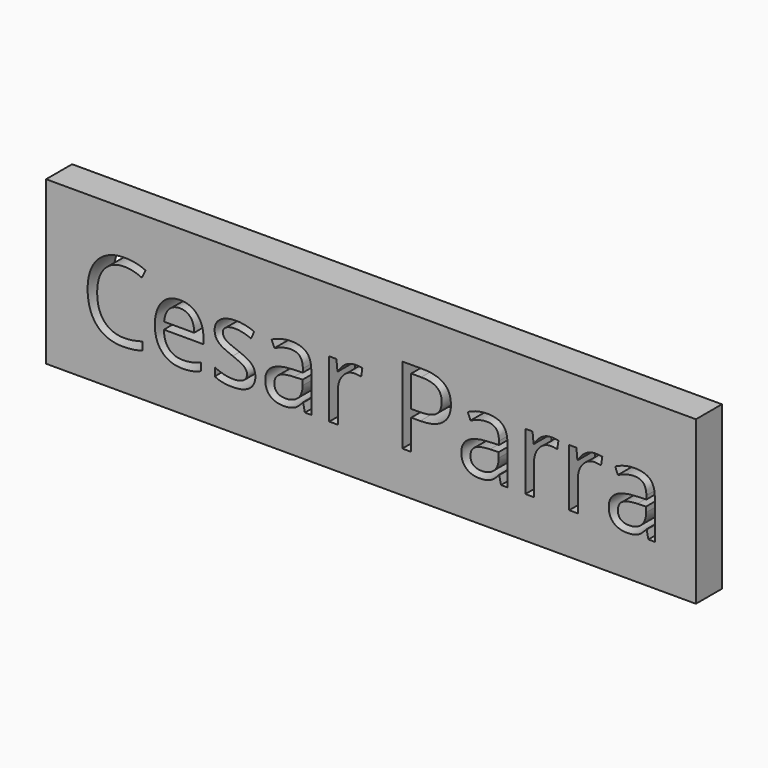
from build123d import *

# Parameters (mm, degrees)
F0_W         = 101.6
F0_H         = 25.4
F1_DEPTH     = 5.08
F2_TEXT_SIZE = 16.7886687753
F3_DEPTH     = 25.4


# Not quite as in the source:
# - Text() gives the source's letters only with a copy of the font that has no kerning and outlines rounded to 1/6400 em; it was checked with that copy


with BuildPart() as f1:
    # F0 (on Front) → F1 (new body)
    with BuildSketch(Plane.XZ):
        with Locations((13.3832387311, 2.4520177394)):
            Rectangle(F0_W, F0_H)
    extrude(amount=F1_DEPTH)

    # F2 (on face) → F3 (cut)
    with BuildSketch(Plane.XZ.offset(5.08)):
        with Locations((-31.9449678063, -3.8109747693)):
            Text('Cesar Parra', F2_TEXT_SIZE, font='Open Sans', text_align=(TextAlign.LEFT, TextAlign.BOTTOM))
    extrude(amount=-F3_DEPTH, mode=Mode.SUBTRACT)


solid = f1.part
